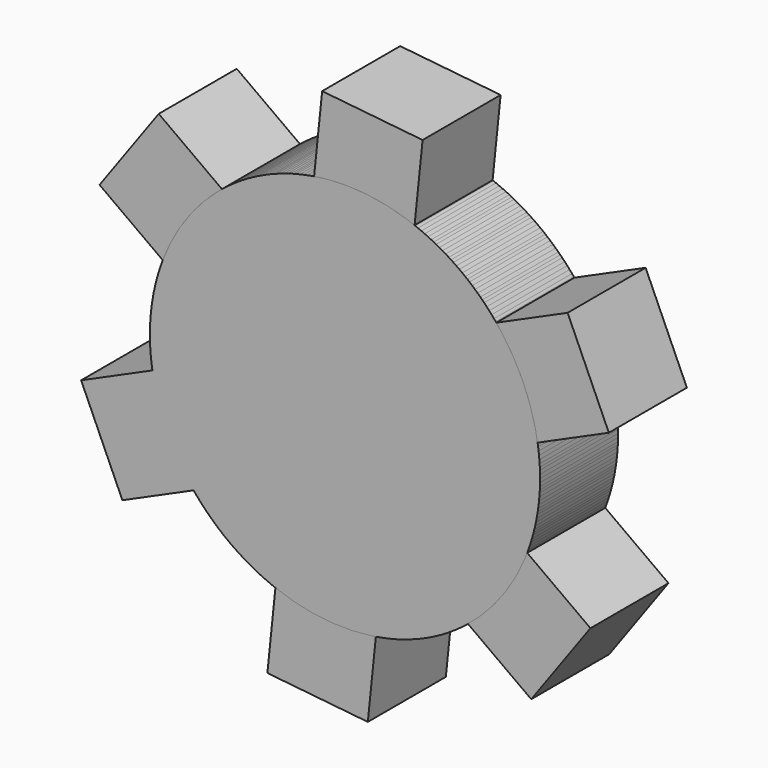
from build123d import *

# Parameters (mm, degrees)
F0_R     = 25.4
F1_DEPTH = 6.35
F3_DEPTH = 12.7
F5_COUNT = 6


# Not quite as in the source:
# - a feature of the source that left no trace in its solid (it failed there, or was rolled back) is left out


with BuildPart() as f1:
    # F0 (on Front) → F1 (new body, symmetric)
    with BuildSketch(Plane.XZ):
        Circle(F0_R)
    extrude(amount=F1_DEPTH, both=True)

    # F2 (on face) → F3 (join)
    with BuildSketch(Plane.XZ.offset(6.35)):
        Polygon((-23.7289304877, 9.0607868263), (0, 0), (-19.8741968407, 14.38606182), align=None)
        Polygon((-19.8741968407, 14.38606182), (0, 0), (-16.0194631938, 19.7113368137), align=None)
        Polygon((-23.7289304877, 9.0607868263), (-19.8741968407, 14.38606182), (-16.0194631938, 19.7113368137), (-24.2495762314, 25.6687556665), (-31.9590435253, 15.0182056791), align=None)
    extrude(amount=-F3_DEPTH)


with BuildPart() as f5_1:
    # F5: instance of F1
    add(f1.part.rotate(Axis((0, 28.0947498977, 0), (0, 1, 0)), 1 * 360 / F5_COUNT))


with BuildPart() as f5_2:
    # F5: instance of F1
    add(f1.part.rotate(Axis((0, 28.0947498977, 0), (0, 1, 0)), 2 * 360 / F5_COUNT))


with BuildPart() as f5_3:
    # F5: instance of F1
    add(f1.part.rotate(Axis((0, 28.0947498977, 0), (0, 1, 0)), 3 * 360 / F5_COUNT))


with BuildPart() as f5_4:
    # F5: instance of F1
    add(f1.part.rotate(Axis((0, 28.0947498977, 0), (0, 1, 0)), 4 * 360 / F5_COUNT))


with BuildPart() as f5_5:
    # F5: instance of F1
    add(f1.part.rotate(Axis((0, 28.0947498977, 0), (0, 1, 0)), 5 * 360 / F5_COUNT))


solid = Compound([f1.part, f5_1.part, f5_2.part, f5_3.part, f5_4.part, f5_5.part])
